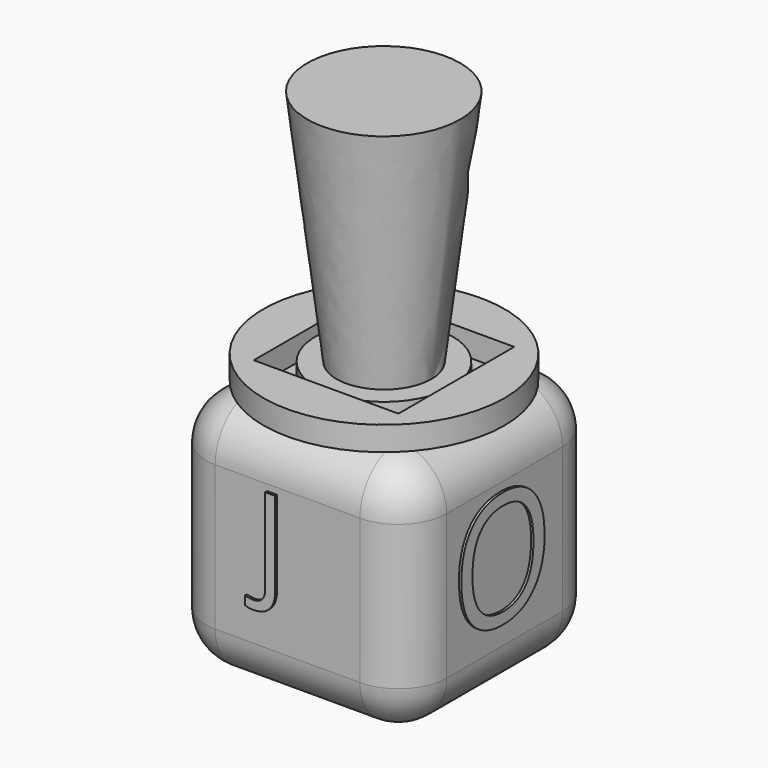
from build123d import *

# Parameters (mm, degrees)
F0_W          = 25.4
F0_H          = 25.4
F1_DEPTH      = 25.4
F2_R          = 5.08
F3_R          = 12.7
F3_W          = 15.24
F3_H          = 15.24
F4_DEPTH      = 2.54
F5_TEXT_SIZE  = 21.1666666667
F6_DEPTH      = 0.25
F7_TEXT_SIZE  = 19.4398071876
F8_DEPTH      = 0.25
F9_TEXT_SIZE  = 12.5475111417
F10_DEPTH     = 0.25
F11_TEXT_SIZE = 16.7005604857
F12_DEPTH     = 0.25
F13_R         = 7.1880698393
F14_DEPTH     = 1.8
F15_R         = 5
F17_R         = 8.0470006945


# Not quite as in the source:
# - Text() gives the source's letters only with a copy of the font that has no kerning and outlines rounded to 1/6400 em; it was checked with that copy


with BuildPart() as f1:
    # F0 (on Front) → F1 (new body)
    with BuildSketch(Plane.XZ):
        with Locations((-32.3449776, 12.7)):
            Rectangle(F0_W, F0_H)
    extrude(amount=F1_DEPTH)

    # F2
    f2_edges = [f1.edges().sort_by_distance(p)[0] for p in [
        (-32.344978, -25.4, 25.4),
        (-19.644978, -12.7, 25.4),
        (-19.644978, -25.4, 12.7),
        (-45.044978, -12.7, 25.4),
        (-32.344978, 0, 25.4),
        (-45.044978, -25.4, 12.7),
        (-32.344978, -25.4, 0),
        (-19.644978, -12.7, 0),
        (-45.044978, -12.7, 0),
        (-32.344978, 0, 0),
        (-19.644978, 0, 12.7),
        (-45.044978, 0, 12.7),
    ]]
    fillet(f2_edges, radius=F2_R)

    # F3 (on face) → F4 (join)
    with BuildSketch(Plane.XY.offset(25.4)):
        with Locations((-32.3449776, -12.7)):
            Circle(F3_R)
        with Locations((-32.3449776, -12.7)):
            Rectangle(F3_W, F3_H, mode=Mode.SUBTRACT)
    extrude(amount=F4_DEPTH)

    # F5 (on face) → F6 (join)
    with BuildSketch(Plane(origin=(0, 0, 0), x_dir=(-1, 0, 0), z_dir=(0, 1, 0))):
        with Locations((27.989274475, 5.08)):
            Text('S', F5_TEXT_SIZE, font='Open Sans', text_align=(TextAlign.LEFT, TextAlign.BOTTOM))
    extrude(amount=F6_DEPTH)

    # F7 (on face) → F8 (join)
    with BuildSketch(Plane(origin=(-45.0449776, 0, 0), x_dir=(0, -1, 0), z_dir=(-1, 0, 0))):
        with Locations((5.6122969836, 5.7274210267)):
            Text('E', F7_TEXT_SIZE, font='Open Sans', text_align=(TextAlign.LEFT, TextAlign.BOTTOM))
    extrude(amount=F8_DEPTH)

    # F9 (on face) → F10 (join)
    with BuildSketch(Plane.XZ.offset(25.4)):
        with Locations((-35.6580205262, 10.6898760423)):
            Text('J', F9_TEXT_SIZE, font='Open Sans', text_align=(TextAlign.LEFT, TextAlign.BOTTOM))
    extrude(amount=F10_DEPTH)

    # F11 (on face) → F12 (join)
    with BuildSketch(Plane.YZ.offset(-19.6449776)):
        with Locations((-19.7301413864, 7.3815723881)):
            Text('O', F11_TEXT_SIZE, font='Open Sans', text_align=(TextAlign.LEFT, TextAlign.BOTTOM))
    extrude(amount=F12_DEPTH)

    # F13 (on face) → F14 (join)
    with BuildSketch(Plane.XY.offset(25.4)):
        with Locations((-32.3449776, -12.7)):
            Circle(F13_R)
    extrude(amount=F14_DEPTH)

    # F15 (on face) → F18 section 0
    with BuildSketch(Plane.XY.offset(27.2)):
        with Locations((-32.3449776, -12.7)):
            Circle(F15_R)
    # F17 (on offset) → F18 section 1
    with BuildSketch(Plane.XY.offset(52.2)):
        with Locations((-32.430421561, -12.6221515238)):
            Circle(F17_R)
    loft()


solid = f1.part
